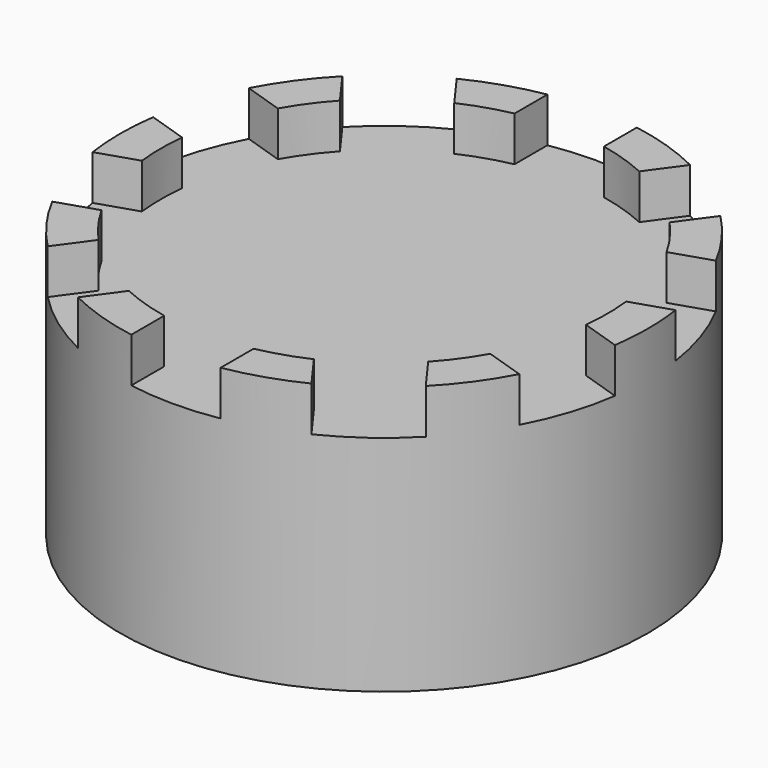
from build123d import *

# Parameters (mm, degrees)
F0_R            = 37.5
F1_DEPTH        = 38.1
F2_W            = 12.7
F2_H            = 12.6999970771
F3_DEPTH        = 37.501
F3_DEPTH_BACK   = 37.501
F3_COPIES_COUNT = 5
F3_COPIES_ANGLE = 144
F5_R            = 31.75
F6_DEPTH        = 6.3509970771


# Not quite as in the source:
# - a pattern or mirror of a feature is missing from the dataset's text; its kind, count and spacing are read off the source's solid


with BuildPart() as f1:
    # F0 (on Top) → F1 (new body)
    with BuildSketch(Plane.XY):
        Circle(F0_R)
    extrude(amount=F1_DEPTH)

    # F2 (on Front) → F3 (cut, two sides)
    with BuildSketch(Plane.XZ) as f3_sk:
        with Locations((0, 38.1000014614)):
            Rectangle(F2_W, F2_H)
    f3 = extrude(amount=F3_DEPTH, mode=Mode.SUBTRACT) + extrude(f3_sk.sketch, amount=-F3_DEPTH_BACK, mode=Mode.SUBTRACT)

    # F3_copies: F3 ×5 about axis
    f3_copies_axis = Axis((0, 0, 0), (0, 0, 1))
    for i in range(1, F3_COPIES_COUNT):
        add(f3.rotate(f3_copies_axis, i * F3_COPIES_ANGLE / (F3_COPIES_COUNT - 1)), mode=Mode.SUBTRACT)

    # F5 (on face) → F6 (cut, through all)
    with BuildSketch(Plane.XY.offset(31.7500029229)):
        Circle(F5_R)
    extrude(amount=F6_DEPTH, mode=Mode.SUBTRACT)


solid = f1.part
